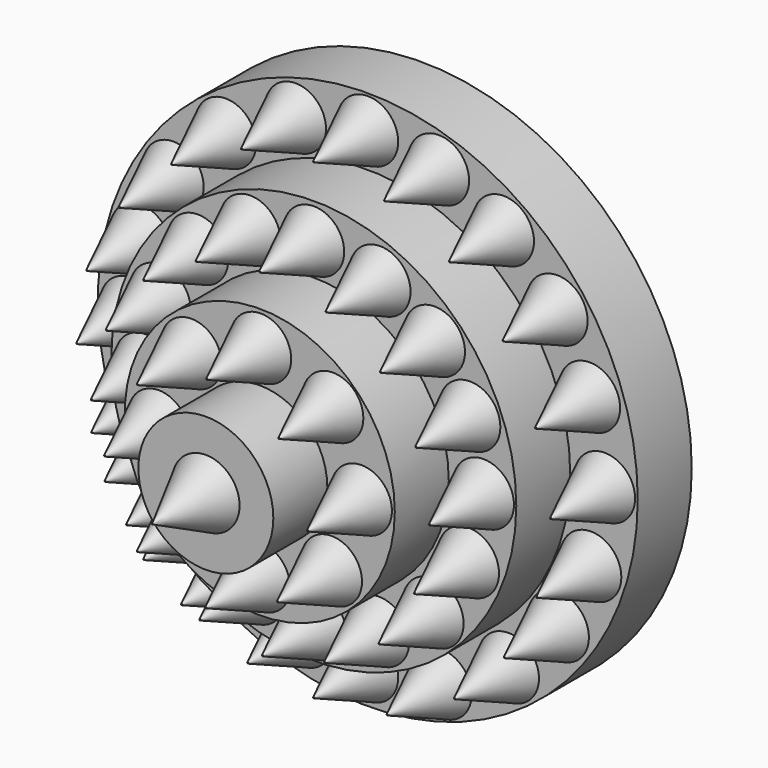
from build123d import *

# Parameters (mm, degrees)
F0_R         = 15.875
F1_DEPTH     = 12.7
F2_R         = 50.8
F3_DEPTH     = 12.7
F4_R         = 38.1
F5_DEPTH     = 12.7
F6_R         = 25.4
F7_DEPTH     = 12.7
F8_R         = 12.7
F9_DEPTH     = 12.7
F10_R        = 6.35
F11_DEPTH    = 12.7
F12_SIZE2    = 12.69999
F12_SIZE     = 6.34999
F13_R        = 5.715
F14_DEPTH    = 12.7
F15_SIZE2    = 12.69999
F15_SIZE     = 5.58799
F15_2_SIZE2  = 12.69999
F15_2_SIZE   = 5.58799
F15_3_SIZE2  = 12.69999
F15_3_SIZE   = 5.58799
F15_4_SIZE2  = 12.69999
F15_4_SIZE   = 5.58799
F15_5_SIZE2  = 12.69999
F15_5_SIZE   = 5.58799
F15_6_SIZE2  = 12.69999
F15_6_SIZE   = 5.58799
F15_7_SIZE2  = 12.69999
F15_7_SIZE   = 5.58799
F15_8_SIZE2  = 12.69999
F15_8_SIZE   = 5.58799
F15_9_SIZE2  = 12.69999
F15_9_SIZE   = 5.58799
F15_10_SIZE2 = 12.69999
F15_10_SIZE  = 5.58799
F15_11_SIZE2 = 12.69999
F15_11_SIZE  = 5.58799
F15_12_SIZE2 = 12.69999
F15_12_SIZE  = 5.58799
F15_13_SIZE2 = 12.69999
F15_13_SIZE  = 5.58799
F15_14_SIZE2 = 12.69999
F15_14_SIZE  = 5.58799
F15_15_SIZE2 = 12.69999
F15_15_SIZE  = 5.58799
F15_16_SIZE2 = 12.69999
F15_16_SIZE  = 5.58799
F15_17_SIZE2 = 12.69999
F15_17_SIZE  = 5.58799
F15_18_SIZE2 = 12.69999
F15_18_SIZE  = 5.58799
F15_19_SIZE2 = 12.69999
F15_19_SIZE  = 5.58799
F15_20_SIZE2 = 12.69999
F15_20_SIZE  = 5.58799
F16_R        = 5.715
F17_DEPTH    = 12.7
F18_SIZE2    = 12.69999
F18_SIZE     = 5.58799
F18_2_SIZE2  = 12.69999
F18_2_SIZE   = 5.58799
F18_3_SIZE2  = 12.69999
F18_3_SIZE   = 5.58799
F18_4_SIZE2  = 12.69999
F18_4_SIZE   = 5.58799
F18_5_SIZE2  = 12.69999
F18_5_SIZE   = 5.58799
F18_6_SIZE2  = 12.69999
F18_6_SIZE   = 5.58799
F18_7_SIZE2  = 12.69999
F18_7_SIZE   = 5.58799
F18_8_SIZE2  = 12.69999
F18_8_SIZE   = 5.58799
F18_9_SIZE2  = 12.69999
F18_9_SIZE   = 5.58799
F18_10_SIZE2 = 12.69999
F18_10_SIZE  = 5.58799
F18_11_SIZE2 = 12.69999
F18_11_SIZE  = 5.58799
F18_12_SIZE2 = 12.69999
F18_12_SIZE  = 5.58799
F18_13_SIZE2 = 12.69999
F18_13_SIZE  = 5.58799
F18_14_SIZE2 = 12.69999
F18_14_SIZE  = 5.58799
F18_15_SIZE2 = 12.69999
F18_15_SIZE  = 5.58799
F18_16_SIZE2 = 12.69999
F18_16_SIZE  = 5.58799
F19_R        = 5.715
F20_DEPTH    = 12.7
F21_SIZE2    = 12.69999
F21_SIZE     = 5.58799
F21_2_SIZE2  = 12.69999
F21_2_SIZE   = 5.58799
F21_3_SIZE2  = 12.69999
F21_3_SIZE   = 5.58799
F21_4_SIZE2  = 12.69999
F21_4_SIZE   = 5.58799
F21_5_SIZE2  = 12.69999
F21_5_SIZE   = 5.58799
F21_6_SIZE2  = 12.69999
F21_6_SIZE   = 5.58799
F21_7_SIZE2  = 12.69999
F21_7_SIZE   = 5.58799
F21_8_SIZE2  = 12.69999
F21_8_SIZE   = 5.58799


# Not quite as in the source:
# - a fillet or chamfer is up to 0.001 mm smaller than in the source, because OpenCascade refuses the exact size


with BuildPart() as f1:
    # F0 (on Front) → F1 (new body)
    with BuildSketch(Plane.XZ):
        Circle(F0_R)
    extrude(amount=F1_DEPTH)

    # F2 (on face) → F3 (join)
    with BuildSketch(Plane.XZ.offset(12.7)):
        Circle(F2_R)
    extrude(amount=F3_DEPTH)

    # F4 (on face) → F5 (join)
    with BuildSketch(Plane.XZ.offset(25.4)):
        Circle(F4_R)
    extrude(amount=F5_DEPTH)

    # F6 (on face) → F7 (join)
    with BuildSketch(Plane.XZ.offset(38.1)):
        Circle(F6_R)
    extrude(amount=F7_DEPTH)

    # F8 (on face) → F9 (join)
    with BuildSketch(Plane.XZ.offset(50.8)):
        Circle(F8_R)
    extrude(amount=F9_DEPTH)

    # F10 (on face) → F11 (join)
    with BuildSketch(Plane.XZ.offset(63.5)):
        Circle(F10_R)
    extrude(amount=F11_DEPTH)

    # F12 (size 6.35 and 12.7 in the source; OpenCascade refuses exactly that, so slightly less here)
    f12_edges = [f1.edges().sort_by_distance(p)[0] for p in [
        (-6.35, -76.2, 0),
    ]]
    f12_side = f1.faces().sort_by_distance((0, -76.2, 0))[0]
    chamfer(f12_edges, length=F12_SIZE, length2=F12_SIZE2, reference=f12_side)

    # F13 (on face) → F14 (join)
    with BuildSketch(Plane.XZ.offset(25.4)):
        with Locations((25.5563743412, 36.3686457276)):
            Circle(F13_R)
        with Locations((35.654515028, 26.505343616)):
            Circle(F13_R)
        with Locations((41.7603701353, 14.0587966889)):
            Circle(F13_R)
        with Locations((44.5784553885, 0)):
            Circle(F13_R)
        with Locations((41.9952087104, -13.8872256503)):
            Circle(F13_R)
        with Locations((35.8893573284, -25.8640907705)):
            Circle(F13_R)
        with Locations((26.4957360923, -35.7273966074)):
            Circle(F13_R)
        with Locations((13.3446659893, 42.4745008349)):
            Circle(F13_R)
        with Locations((0, 44.5880666375)):
            Circle(F13_R)
        with Locations((0, -44.1816560924)):
            Circle(F13_R)
        with Locations((13.8143477961, -42.5377674401)):
            Circle(F13_R)
        with Locations((-12.4053042382, -42.4745008349)):
            Circle(F13_R)
        with Locations((-24.8518530279, -36.8383266032)):
            Circle(F13_R)
        with Locations((-35.1848341525, -26.9750244915)):
            Circle(F13_R)
        with Locations((-41.7603701353, -13.8239562511)):
            Circle(F13_R)
        with Locations((-44.5784553885, 0)):
            Circle(F13_R)
        with Locations((-42.6997318864, 12.7130225301)):
            Circle(F13_R)
        with Locations((-36.5938767791, 25.1595713198)):
            Circle(F13_R)
        with Locations((-26.7305765301, 35.492554307)):
            Circle(F13_R)
        with Locations((-13.579506427, 42.3029251397)):
            Circle(F13_R)
    extrude(amount=F14_DEPTH)

    # F15 (size 5.588 and 12.7 in the source; OpenCascade refuses exactly that, so slightly less here)
    f15_edges = [f1.edges().sort_by_distance(p)[0] for p in [
        (-47.47537, -38.1, -13.823956),
    ]]
    f15_side = f1.faces().sort_by_distance((-41.76037, -38.1, -13.823956))[0]
    chamfer(f15_edges, length=F15_SIZE, length2=F15_SIZE2, reference=f15_side)

    # F15#2 (size 5.588 and 12.7 in the source; OpenCascade refuses exactly that, so slightly less here)
    f15_2_edges = [f1.edges().sort_by_distance(p)[0] for p in [
        (-50.293455, -38.1, 0),
    ]]
    f15_2_side = f1.faces().sort_by_distance((-44.578455, -38.1, 0))[0]
    chamfer(f15_2_edges, length=F15_2_SIZE, length2=F15_2_SIZE2, reference=f15_2_side)

    # F15#3 (size 5.588 and 12.7 in the source; OpenCascade refuses exactly that, so slightly less here)
    f15_3_edges = [f1.edges().sort_by_distance(p)[0] for p in [
        (-48.414732, -38.1, 12.713023),
    ]]
    f15_3_side = f1.faces().sort_by_distance((-42.699732, -38.1, 12.713023))[0]
    chamfer(f15_3_edges, length=F15_3_SIZE, length2=F15_3_SIZE2, reference=f15_3_side)

    # F15#4 (size 5.588 and 12.7 in the source; OpenCascade refuses exactly that, so slightly less here)
    f15_4_edges = [f1.edges().sort_by_distance(p)[0] for p in [
        (-42.308877, -38.1, 25.159571),
    ]]
    f15_4_side = f1.faces().sort_by_distance((-36.593877, -38.1, 25.159571))[0]
    chamfer(f15_4_edges, length=F15_4_SIZE, length2=F15_4_SIZE2, reference=f15_4_side)

    # F15#5 (size 5.588 and 12.7 in the source; OpenCascade refuses exactly that, so slightly less here)
    f15_5_edges = [f1.edges().sort_by_distance(p)[0] for p in [
        (-32.445577, -38.1, 35.492554),
    ]]
    f15_5_side = f1.faces().sort_by_distance((-26.730577, -38.1, 35.492554))[0]
    chamfer(f15_5_edges, length=F15_5_SIZE, length2=F15_5_SIZE2, reference=f15_5_side)

    # F15#6 (size 5.588 and 12.7 in the source; OpenCascade refuses exactly that, so slightly less here)
    f15_6_edges = [f1.edges().sort_by_distance(p)[0] for p in [
        (-19.294506, -38.1, 42.302925),
    ]]
    f15_6_side = f1.faces().sort_by_distance((-13.579506, -38.1, 42.302925))[0]
    chamfer(f15_6_edges, length=F15_6_SIZE, length2=F15_6_SIZE2, reference=f15_6_side)

    # F15#7 (size 5.588 and 12.7 in the source; OpenCascade refuses exactly that, so slightly less here)
    f15_7_edges = [f1.edges().sort_by_distance(p)[0] for p in [
        (-5.715, -38.1, 44.588067),
    ]]
    f15_7_side = f1.faces().sort_by_distance((0, -38.1, 44.588067))[0]
    chamfer(f15_7_edges, length=F15_7_SIZE, length2=F15_7_SIZE2, reference=f15_7_side)

    # F15#8 (size 5.588 and 12.7 in the source; OpenCascade refuses exactly that, so slightly less here)
    f15_8_edges = [f1.edges().sort_by_distance(p)[0] for p in [
        (7.629666, -38.1, 42.474501),
    ]]
    f15_8_side = f1.faces().sort_by_distance((13.344666, -38.1, 42.474501))[0]
    chamfer(f15_8_edges, length=F15_8_SIZE, length2=F15_8_SIZE2, reference=f15_8_side)

    # F15#9 (size 5.588 and 12.7 in the source; OpenCascade refuses exactly that, so slightly less here)
    f15_9_edges = [f1.edges().sort_by_distance(p)[0] for p in [
        (19.841374, -38.1, 36.368646),
    ]]
    f15_9_side = f1.faces().sort_by_distance((25.556374, -38.1, 36.368646))[0]
    chamfer(f15_9_edges, length=F15_9_SIZE, length2=F15_9_SIZE2, reference=f15_9_side)

    # F15#10 (size 5.588 and 12.7 in the source; OpenCascade refuses exactly that, so slightly less here)
    f15_10_edges = [f1.edges().sort_by_distance(p)[0] for p in [
        (29.939515, -38.1, 26.505344),
    ]]
    f15_10_side = f1.faces().sort_by_distance((35.654515, -38.1, 26.505344))[0]
    chamfer(f15_10_edges, length=F15_10_SIZE, length2=F15_10_SIZE2, reference=f15_10_side)

    # F15#11 (size 5.588 and 12.7 in the source; OpenCascade refuses exactly that, so slightly less here)
    f15_11_edges = [f1.edges().sort_by_distance(p)[0] for p in [
        (36.04537, -38.1, 14.058797),
    ]]
    f15_11_side = f1.faces().sort_by_distance((41.76037, -38.1, 14.058797))[0]
    chamfer(f15_11_edges, length=F15_11_SIZE, length2=F15_11_SIZE2, reference=f15_11_side)

    # F15#12 (size 5.588 and 12.7 in the source; OpenCascade refuses exactly that, so slightly less here)
    f15_12_edges = [f1.edges().sort_by_distance(p)[0] for p in [
        (38.863455, -38.1, 0),
    ]]
    f15_12_side = f1.faces().sort_by_distance((44.578455, -38.1, 0))[0]
    chamfer(f15_12_edges, length=F15_12_SIZE, length2=F15_12_SIZE2, reference=f15_12_side)

    # F15#13 (size 5.588 and 12.7 in the source; OpenCascade refuses exactly that, so slightly less here)
    f15_13_edges = [f1.edges().sort_by_distance(p)[0] for p in [
        (36.280209, -38.1, -13.887226),
    ]]
    f15_13_side = f1.faces().sort_by_distance((41.995209, -38.1, -13.887226))[0]
    chamfer(f15_13_edges, length=F15_13_SIZE, length2=F15_13_SIZE2, reference=f15_13_side)

    # F15#14 (size 5.588 and 12.7 in the source; OpenCascade refuses exactly that, so slightly less here)
    f15_14_edges = [f1.edges().sort_by_distance(p)[0] for p in [
        (30.174357, -38.1, -25.864091),
    ]]
    f15_14_side = f1.faces().sort_by_distance((35.889357, -38.1, -25.864091))[0]
    chamfer(f15_14_edges, length=F15_14_SIZE, length2=F15_14_SIZE2, reference=f15_14_side)

    # F15#15 (size 5.588 and 12.7 in the source; OpenCascade refuses exactly that, so slightly less here)
    f15_15_edges = [f1.edges().sort_by_distance(p)[0] for p in [
        (20.780736, -38.1, -35.727397),
    ]]
    f15_15_side = f1.faces().sort_by_distance((26.495736, -38.1, -35.727397))[0]
    chamfer(f15_15_edges, length=F15_15_SIZE, length2=F15_15_SIZE2, reference=f15_15_side)

    # F15#16 (size 5.588 and 12.7 in the source; OpenCascade refuses exactly that, so slightly less here)
    f15_16_edges = [f1.edges().sort_by_distance(p)[0] for p in [
        (8.099348, -38.1, -42.537767),
    ]]
    f15_16_side = f1.faces().sort_by_distance((13.814348, -38.1, -42.537767))[0]
    chamfer(f15_16_edges, length=F15_16_SIZE, length2=F15_16_SIZE2, reference=f15_16_side)

    # F15#17 (size 5.588 and 12.7 in the source; OpenCascade refuses exactly that, so slightly less here)
    f15_17_edges = [f1.edges().sort_by_distance(p)[0] for p in [
        (-5.715, -38.1, -44.181656),
    ]]
    f15_17_side = f1.faces().sort_by_distance((0, -38.1, -44.181656))[0]
    chamfer(f15_17_edges, length=F15_17_SIZE, length2=F15_17_SIZE2, reference=f15_17_side)

    # F15#18 (size 5.588 and 12.7 in the source; OpenCascade refuses exactly that, so slightly less here)
    f15_18_edges = [f1.edges().sort_by_distance(p)[0] for p in [
        (-18.120304, -38.1, -42.474501),
    ]]
    f15_18_side = f1.faces().sort_by_distance((-12.405304, -38.1, -42.474501))[0]
    chamfer(f15_18_edges, length=F15_18_SIZE, length2=F15_18_SIZE2, reference=f15_18_side)

    # F15#19 (size 5.588 and 12.7 in the source; OpenCascade refuses exactly that, so slightly less here)
    f15_19_edges = [f1.edges().sort_by_distance(p)[0] for p in [
        (-30.566853, -38.1, -36.838327),
    ]]
    f15_19_side = f1.faces().sort_by_distance((-24.851853, -38.1, -36.838327))[0]
    chamfer(f15_19_edges, length=F15_19_SIZE, length2=F15_19_SIZE2, reference=f15_19_side)

    # F15#20 (size 5.588 and 12.7 in the source; OpenCascade refuses exactly that, so slightly less here)
    f15_20_edges = [f1.edges().sort_by_distance(p)[0] for p in [
        (-40.899834, -38.1, -26.975024),
    ]]
    f15_20_side = f1.faces().sort_by_distance((-35.184834, -38.1, -26.975024))[0]
    chamfer(f15_20_edges, length=F15_20_SIZE, length2=F15_20_SIZE2, reference=f15_20_side)

    # F16 (on face) → F17 (join)
    with BuildSketch(Plane.XZ.offset(38.1)):
        with Locations((-31.682536006, 0)):
            Circle(F16_R)
        with Locations((0, 31.5002650023)):
            Circle(F16_R)
        with Locations((0.5109232152, -31.9066755474)):
            Circle(F16_R)
        with Locations((31.9478400052, 0)):
            Circle(F16_R)
        with Locations((29.3868873268, 12.0437536389)):
            Circle(F16_R)
        with Locations((22.7284058928, 22.2875680774)):
            Circle(F16_R)
        with Locations((12.4845905229, 28.9460495114)):
            Circle(F16_R)
        with Locations((29.1307903826, -12.2853098437)):
            Circle(F16_R)
        with Locations((22.4723108113, -22.7852221578)):
            Circle(F16_R)
        with Locations((12.2284954414, -29.1876066476)):
            Circle(F16_R)
        with Locations((-11.2514095381, -29.7931116074)):
            Circle(F16_R)
        with Locations((-21.8192338943, -23.2175774872)):
            Circle(F16_R)
        with Locations((-29.0992893279, -12.649753131)):
            Circle(F16_R)
        with Locations((-28.8644488901, 12.4781830236)):
            Circle(F16_R)
        with Locations((-21.8192338943, 23.0460055172)):
            Circle(F16_R)
        with Locations((-11.9559308514, 29.3867010623)):
            Circle(F16_R)
    extrude(amount=F17_DEPTH)

    # F18 (size 5.588 and 12.7 in the source; OpenCascade refuses exactly that, so slightly less here)
    f18_edges = [f1.edges().sort_by_distance(p)[0] for p in [
        (23.41579, -50.8, -12.28531),
    ]]
    f18_side = f1.faces().sort_by_distance((29.13079, -50.8, -12.28531))[0]
    chamfer(f18_edges, length=F18_SIZE, length2=F18_SIZE2, reference=f18_side)

    # F18#2 (size 5.588 and 12.7 in the source; OpenCascade refuses exactly that, so slightly less here)
    f18_2_edges = [f1.edges().sort_by_distance(p)[0] for p in [
        (26.23284, -50.8, 0),
    ]]
    f18_2_side = f1.faces().sort_by_distance((31.94784, -50.8, 0))[0]
    chamfer(f18_2_edges, length=F18_2_SIZE, length2=F18_2_SIZE2, reference=f18_2_side)

    # F18#3 (size 5.588 and 12.7 in the source; OpenCascade refuses exactly that, so slightly less here)
    f18_3_edges = [f1.edges().sort_by_distance(p)[0] for p in [
        (23.671887, -50.8, 12.043754),
    ]]
    f18_3_side = f1.faces().sort_by_distance((29.386887, -50.8, 12.043754))[0]
    chamfer(f18_3_edges, length=F18_3_SIZE, length2=F18_3_SIZE2, reference=f18_3_side)

    # F18#4 (size 5.588 and 12.7 in the source; OpenCascade refuses exactly that, so slightly less here)
    f18_4_edges = [f1.edges().sort_by_distance(p)[0] for p in [
        (17.013406, -50.8, 22.287568),
    ]]
    f18_4_side = f1.faces().sort_by_distance((22.728406, -50.8, 22.287568))[0]
    chamfer(f18_4_edges, length=F18_4_SIZE, length2=F18_4_SIZE2, reference=f18_4_side)

    # F18#5 (size 5.588 and 12.7 in the source; OpenCascade refuses exactly that, so slightly less here)
    f18_5_edges = [f1.edges().sort_by_distance(p)[0] for p in [
        (6.769591, -50.8, 28.94605),
    ]]
    f18_5_side = f1.faces().sort_by_distance((12.484591, -50.8, 28.94605))[0]
    chamfer(f18_5_edges, length=F18_5_SIZE, length2=F18_5_SIZE2, reference=f18_5_side)

    # F18#6 (size 5.588 and 12.7 in the source; OpenCascade refuses exactly that, so slightly less here)
    f18_6_edges = [f1.edges().sort_by_distance(p)[0] for p in [
        (-5.715, -50.8, 31.500265),
    ]]
    f18_6_side = f1.faces().sort_by_distance((0, -50.8, 31.500265))[0]
    chamfer(f18_6_edges, length=F18_6_SIZE, length2=F18_6_SIZE2, reference=f18_6_side)

    # F18#7 (size 5.588 and 12.7 in the source; OpenCascade refuses exactly that, so slightly less here)
    f18_7_edges = [f1.edges().sort_by_distance(p)[0] for p in [
        (-17.670931, -50.8, 29.386701),
    ]]
    f18_7_side = f1.faces().sort_by_distance((-11.955931, -50.8, 29.386701))[0]
    chamfer(f18_7_edges, length=F18_7_SIZE, length2=F18_7_SIZE2, reference=f18_7_side)

    # F18#8 (size 5.588 and 12.7 in the source; OpenCascade refuses exactly that, so slightly less here)
    f18_8_edges = [f1.edges().sort_by_distance(p)[0] for p in [
        (-27.534234, -50.8, 23.046006),
    ]]
    f18_8_side = f1.faces().sort_by_distance((-21.819234, -50.8, 23.046006))[0]
    chamfer(f18_8_edges, length=F18_8_SIZE, length2=F18_8_SIZE2, reference=f18_8_side)

    # F18#9 (size 5.588 and 12.7 in the source; OpenCascade refuses exactly that, so slightly less here)
    f18_9_edges = [f1.edges().sort_by_distance(p)[0] for p in [
        (-34.579449, -50.8, 12.478183),
    ]]
    f18_9_side = f1.faces().sort_by_distance((-28.864449, -50.8, 12.478183))[0]
    chamfer(f18_9_edges, length=F18_9_SIZE, length2=F18_9_SIZE2, reference=f18_9_side)

    # F18#10 (size 5.588 and 12.7 in the source; OpenCascade refuses exactly that, so slightly less here)
    f18_10_edges = [f1.edges().sort_by_distance(p)[0] for p in [
        (-37.397536, -50.8, 0),
    ]]
    f18_10_side = f1.faces().sort_by_distance((-31.682536, -50.8, 0))[0]
    chamfer(f18_10_edges, length=F18_10_SIZE, length2=F18_10_SIZE2, reference=f18_10_side)

    # F18#11 (size 5.588 and 12.7 in the source; OpenCascade refuses exactly that, so slightly less here)
    f18_11_edges = [f1.edges().sort_by_distance(p)[0] for p in [
        (-34.814289, -50.8, -12.649753),
    ]]
    f18_11_side = f1.faces().sort_by_distance((-29.099289, -50.8, -12.649753))[0]
    chamfer(f18_11_edges, length=F18_11_SIZE, length2=F18_11_SIZE2, reference=f18_11_side)

    # F18#12 (size 5.588 and 12.7 in the source; OpenCascade refuses exactly that, so slightly less here)
    f18_12_edges = [f1.edges().sort_by_distance(p)[0] for p in [
        (-27.534234, -50.8, -23.217577),
    ]]
    f18_12_side = f1.faces().sort_by_distance((-21.819234, -50.8, -23.217577))[0]
    chamfer(f18_12_edges, length=F18_12_SIZE, length2=F18_12_SIZE2, reference=f18_12_side)

    # F18#13 (size 5.588 and 12.7 in the source; OpenCascade refuses exactly that, so slightly less here)
    f18_13_edges = [f1.edges().sort_by_distance(p)[0] for p in [
        (-16.96641, -50.8, -29.793112),
    ]]
    f18_13_side = f1.faces().sort_by_distance((-11.25141, -50.8, -29.793112))[0]
    chamfer(f18_13_edges, length=F18_13_SIZE, length2=F18_13_SIZE2, reference=f18_13_side)

    # F18#14 (size 5.588 and 12.7 in the source; OpenCascade refuses exactly that, so slightly less here)
    f18_14_edges = [f1.edges().sort_by_distance(p)[0] for p in [
        (-5.204077, -50.8, -31.906676),
    ]]
    f18_14_side = f1.faces().sort_by_distance((0.510923, -50.8, -31.906676))[0]
    chamfer(f18_14_edges, length=F18_14_SIZE, length2=F18_14_SIZE2, reference=f18_14_side)

    # F18#15 (size 5.588 and 12.7 in the source; OpenCascade refuses exactly that, so slightly less here)
    f18_15_edges = [f1.edges().sort_by_distance(p)[0] for p in [
        (6.513495, -50.8, -29.187607),
    ]]
    f18_15_side = f1.faces().sort_by_distance((12.228495, -50.8, -29.187607))[0]
    chamfer(f18_15_edges, length=F18_15_SIZE, length2=F18_15_SIZE2, reference=f18_15_side)

    # F18#16 (size 5.588 and 12.7 in the source; OpenCascade refuses exactly that, so slightly less here)
    f18_16_edges = [f1.edges().sort_by_distance(p)[0] for p in [
        (16.757311, -50.8, -22.785222),
    ]]
    f18_16_side = f1.faces().sort_by_distance((22.472311, -50.8, -22.785222))[0]
    chamfer(f18_16_edges, length=F18_16_SIZE, length2=F18_16_SIZE2, reference=f18_16_side)

    # F19 (on face) → F20 (join)
    with BuildSketch(Plane.XZ.offset(50.8)):
        with Locations((-19.0151426941, 0)):
            Circle(F19_R)
        with Locations((0.1920116483, 18.9583282918)):
            Circle(F19_R)
        with Locations((19.1430710256, 0)):
            Circle(F19_R)
        with Locations((0, -18.9437903464)):
            Circle(F19_R)
        with Locations((-12.8688542172, -13.8218821958)):
            Circle(F19_R)
        with Locations((-12.8688542172, 13.8364220038)):
            Circle(F19_R)
        with Locations((13.7650659308, 13.5803259909)):
            Circle(F19_R)
        with Locations((13.5089717805, -13.5657871142)):
            Circle(F19_R)
    extrude(amount=F20_DEPTH)

    # F21 (size 5.588 and 12.7 in the source; OpenCascade refuses exactly that, so slightly less here)
    f21_edges = [f1.edges().sort_by_distance(p)[0] for p in [
        (-5.715, -63.5, -18.94379),
    ]]
    f21_side = f1.faces().sort_by_distance((0, -63.5, -18.94379))[0]
    chamfer(f21_edges, length=F21_SIZE, length2=F21_SIZE2, reference=f21_side)

    # F21#2 (size 5.588 and 12.7 in the source; OpenCascade refuses exactly that, so slightly less here)
    f21_2_edges = [f1.edges().sort_by_distance(p)[0] for p in [
        (-18.583854, -63.5, -13.821882),
    ]]
    f21_2_side = f1.faces().sort_by_distance((-12.868854, -63.5, -13.821882))[0]
    chamfer(f21_2_edges, length=F21_2_SIZE, length2=F21_2_SIZE2, reference=f21_2_side)

    # F21#3 (size 5.588 and 12.7 in the source; OpenCascade refuses exactly that, so slightly less here)
    f21_3_edges = [f1.edges().sort_by_distance(p)[0] for p in [
        (-24.730143, -63.5, 0),
    ]]
    f21_3_side = f1.faces().sort_by_distance((-19.015143, -63.5, 0))[0]
    chamfer(f21_3_edges, length=F21_3_SIZE, length2=F21_3_SIZE2, reference=f21_3_side)

    # F21#4 (size 5.588 and 12.7 in the source; OpenCascade refuses exactly that, so slightly less here)
    f21_4_edges = [f1.edges().sort_by_distance(p)[0] for p in [
        (-18.583854, -63.5, 13.836422),
    ]]
    f21_4_side = f1.faces().sort_by_distance((-12.868854, -63.5, 13.836422))[0]
    chamfer(f21_4_edges, length=F21_4_SIZE, length2=F21_4_SIZE2, reference=f21_4_side)

    # F21#5 (size 5.588 and 12.7 in the source; OpenCascade refuses exactly that, so slightly less here)
    f21_5_edges = [f1.edges().sort_by_distance(p)[0] for p in [
        (-5.522988, -63.5, 18.958328),
    ]]
    f21_5_side = f1.faces().sort_by_distance((0.192012, -63.5, 18.958328))[0]
    chamfer(f21_5_edges, length=F21_5_SIZE, length2=F21_5_SIZE2, reference=f21_5_side)

    # F21#6 (size 5.588 and 12.7 in the source; OpenCascade refuses exactly that, so slightly less here)
    f21_6_edges = [f1.edges().sort_by_distance(p)[0] for p in [
        (8.050066, -63.5, 13.580326),
    ]]
    f21_6_side = f1.faces().sort_by_distance((13.765066, -63.5, 13.580326))[0]
    chamfer(f21_6_edges, length=F21_6_SIZE, length2=F21_6_SIZE2, reference=f21_6_side)

    # F21#7 (size 5.588 and 12.7 in the source; OpenCascade refuses exactly that, so slightly less here)
    f21_7_edges = [f1.edges().sort_by_distance(p)[0] for p in [
        (13.428071, -63.5, 0),
    ]]
    f21_7_side = f1.faces().sort_by_distance((19.143071, -63.5, 0))[0]
    chamfer(f21_7_edges, length=F21_7_SIZE, length2=F21_7_SIZE2, reference=f21_7_side)

    # F21#8 (size 5.588 and 12.7 in the source; OpenCascade refuses exactly that, so slightly less here)
    f21_8_edges = [f1.edges().sort_by_distance(p)[0] for p in [
        (7.793972, -63.5, -13.565787),
    ]]
    f21_8_side = f1.faces().sort_by_distance((13.508972, -63.5, -13.565787))[0]
    chamfer(f21_8_edges, length=F21_8_SIZE, length2=F21_8_SIZE2, reference=f21_8_side)


solid = f1.part
